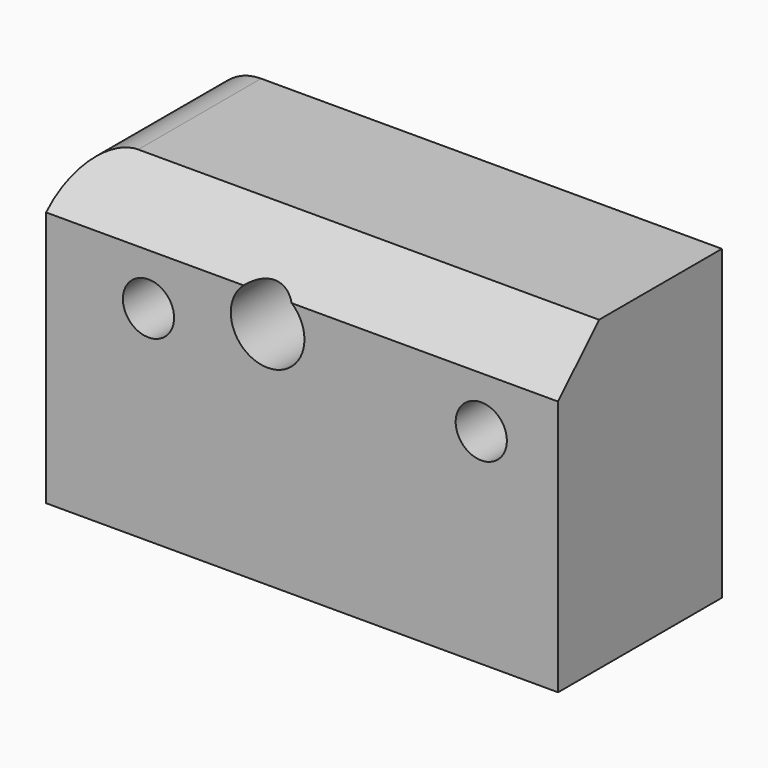
from build123d import *

# Parameters (mm, degrees)
F0_W        = 127
F0_H        = 76.2
F0_R        = 6.35
F1_DEPTH    = 50.8
F2_R        = 9.1340050973
F3_DEPTH    = 70.104
F4_T1_DEPTH = 192.3207478943
F5_R        = 12.7


# Not quite as in the source:
# - a fillet or chamfer that OpenCascade refuses, or shapes differently, is made with other operations: its cross-section is extruded or revolved along the edge and cut away or added


with BuildPart() as f1:
    # F0 (on Front) → F1 (new body)
    with BuildSketch(Plane.XZ):
        with Locations((4.9776248634, -39.8979571181)):
            Rectangle(F0_W, F0_H)
        with Locations((-33.1223751366, -27.1979571181)):
            Circle(F0_R, mode=Mode.SUBTRACT)
        with Locations((49.4276248634, -27.1979571181)):
            Circle(F0_R, mode=Mode.SUBTRACT)
    extrude(amount=F1_DEPTH)

    # F2 (on face) → F3 (cut)
    with BuildSketch(Plane.XZ.offset(50.8)):
        with Locations((-3.571436042, -21.4178189635)):
            Circle(F2_R)
    extrude(amount=-F3_DEPTH, mode=Mode.SUBTRACT)

    # F4: chamfer of 12.7 on 1 edges, made by hand

    # F4_s2 → F4_t1 (cut)
    with BuildSketch(Plane.YZ.offset(-91.1827490838)):
        Polygon((-38.1, -1.7979571181), (-50.8, -14.4979571181), (-50.8, -1.7979571181), align=None)
    extrude(amount=F4_T1_DEPTH, mode=Mode.SUBTRACT)

    # F5
    f5_edges = [f1.edges().sort_by_distance(p)[0] for p in [
        (-58.522375, -19.05, -1.797957),
    ]]
    fillet(f5_edges, radius=F5_R)


solid = f1.part
